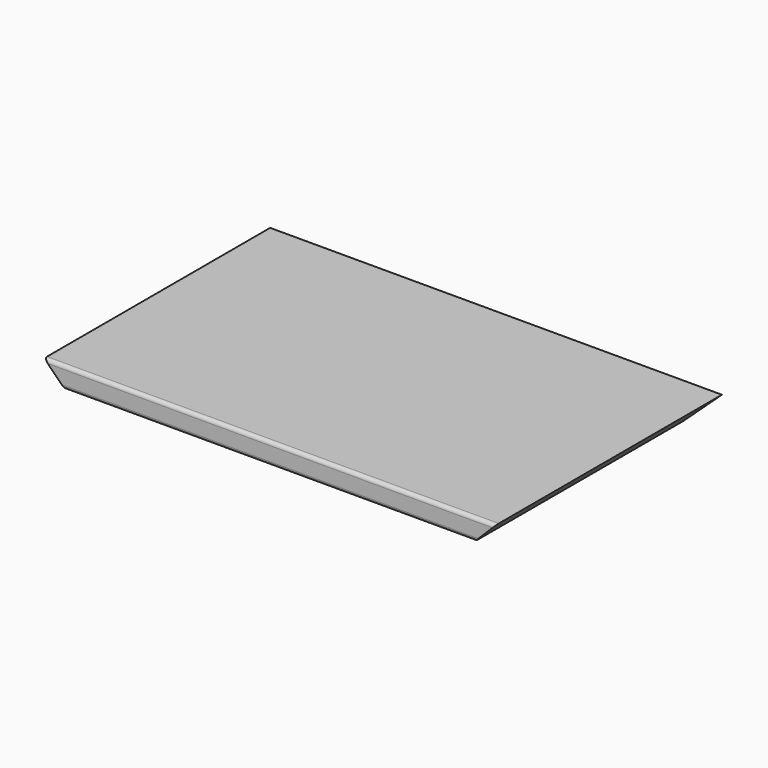
from build123d import *

# Parameters (mm, degrees)
F1_DEPTH = 254
F2_SIZE  = 19.04999
F3_W     = 63.5
F3_H     = 19.05
F4_DEPTH = 6.35
F5_R     = 3.175


# Not quite as in the source:
# - a fillet or chamfer is up to 0.001 mm smaller than in the source, because OpenCascade refuses the exact size


with BuildPart() as f1:
    # F0 (on Front) → F1 (new body)
    with BuildSketch(Plane.XZ):
        Polygon((203.2, 9.525), (-203.2, 9.525), (-184.15, -9.525), (184.15, -9.525), align=None)
    extrude(amount=-F1_DEPTH)

    # F2 (size 19.05 in the source; OpenCascade refuses exactly that, so slightly less here)
    f2_edges = [f1.edges().sort_by_distance(p)[0] for p in [
        (0, 254, -9.525),
    ]]
    chamfer(f2_edges, length=F2_SIZE)

    # F3 (on face) → F4 (cut)
    with BuildSketch(Plane(origin=(0, 0, -9.525), x_dir=(1, 0, 0), z_dir=(0, 0, -1))):
        with Locations((-152.4, -28.575)):
            Rectangle(F3_W, F3_H)
        with Locations((31.75, -28.575)):
            Rectangle(F3_W, F3_H)
        with Locations((31.75, -206.375)):
            Rectangle(F3_W, F3_H)
        with Locations((-152.4, -206.375)):
            Rectangle(F3_W, F3_H)
    extrude(amount=-F4_DEPTH, mode=Mode.SUBTRACT)

    # F5
    f5_edges = [f1.edges().sort_by_distance(p)[0] for p in [
        (0, 0, 9.525),
        (0, 0, -9.525),
    ]]
    fillet(f5_edges, radius=F5_R)


solid = f1.part
